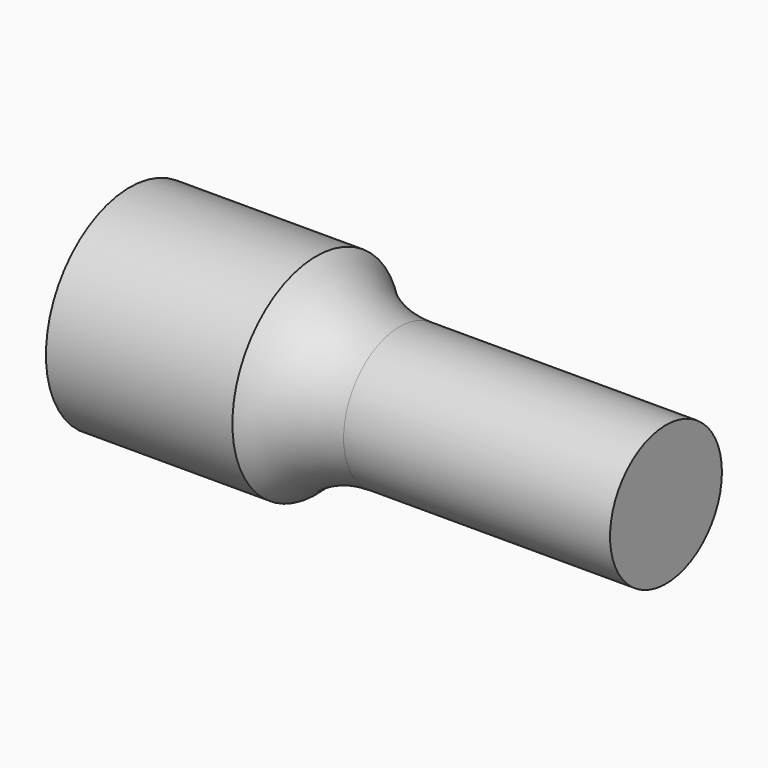
from build123d import *


# Not quite as in the source:
# - a fillet or chamfer that OpenCascade refuses, or shapes differently, is made with other operations: its cross-section is extruded or revolved along the edge and cut away or added


with BuildPart() as f1:
    # F0 (on Top) → F1 (revolve)
    with BuildSketch(Plane.XY):
        Polygon((-11.5, 4.5), (-11.5, 0), (11.5, 0), (11.5, 3), (-3.5, 3), (-3.5, 4.5), align=None)
    revolve(axis=Axis((-2.8623924786, 0, 0), (1, 0, 0)))

    # F2: fillet of radius 5 on 1 edges, made by hand

    # F2_s1 → F2_t2 (revolve)
    with BuildSketch(Plane.XY):
        with BuildLine():
            ThreePointArc((0.0707142143, 3), (-1.8657774588, 3.3902277714), (-3.5, 4.5))
            Line((-3.5, 4.5), (-3.5, 3))
            Line((-3.5, 3), (0.0707142143, 3))
        make_face()
    revolve(axis=Axis((-3.5, 0, 0), (1, 0, 0)))


solid = f1.part
